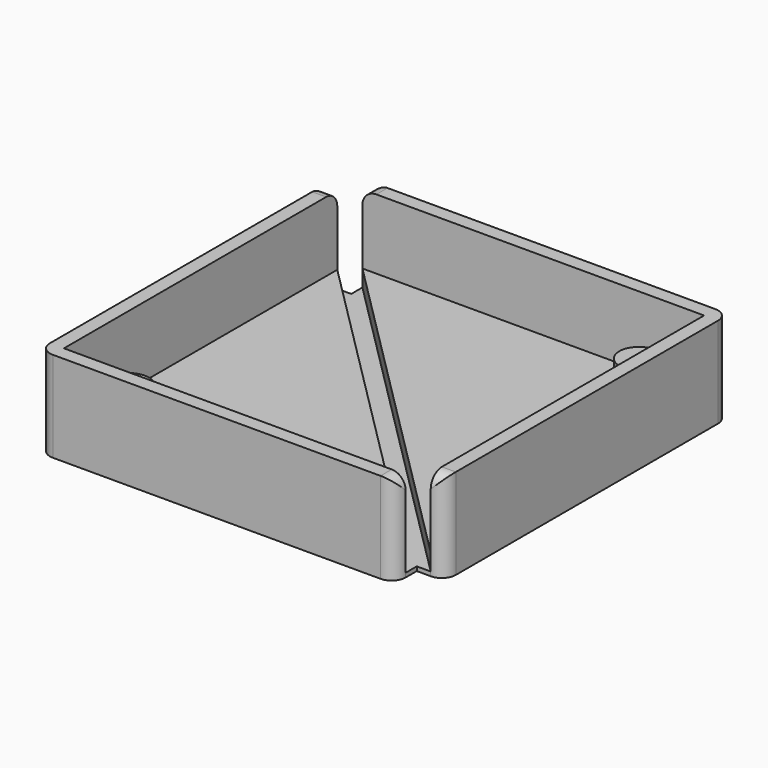
from build123d import *

# Parameters (mm, degrees)
F0_W     = 55
F0_H     = 55
F1_DEPTH = 3
F2_W     = 55
F2_H     = 55
F2_W_2   = 51
F2_H_2   = 51
F3_DEPTH = 10
F4_R     = 2.8
F5_DEPTH = 5
F6_W     = 4
F6_H     = 4
F7_DEPTH = 25
F9_DEPTH = 2.4
F10_R    = 1.99999


# Not quite as in the source:
# - a fillet or chamfer is up to 0.001 mm smaller than in the source, because OpenCascade refuses the exact size


with BuildPart() as f1:
    # F0 (on Top) → F1 (new body)
    with BuildSketch(Plane.XY):
        Rectangle(F0_W, F0_H)
    extrude(amount=F1_DEPTH)

    # F2 (on face) → F3 (join)
    with BuildSketch(Plane.XY.offset(3)):
        Rectangle(F2_W, F2_H)
        Rectangle(F2_W_2, F2_H_2, mode=Mode.SUBTRACT)
    extrude(amount=F3_DEPTH)

    # F4 (on face) → F5 (join)
    with BuildSketch(Plane.XY.offset(3)):
        with Locations((-20.3, -20.3)):
            Circle(F4_R)
        with Locations((20.3, 20.3)):
            Circle(F4_R)
    extrude(amount=F5_DEPTH)

    # F6 (on face) → F7 (cut)
    with BuildSketch(Plane.XY.offset(13)):
        with Locations((-25.5, 25.5)):
            Rectangle(F6_W, F6_H)
        with Locations((25.5, -25.5)):
            Rectangle(F6_W, F6_H)
    extrude(amount=-F7_DEPTH, mode=Mode.SUBTRACT)

    # F8 (on face) → F9 (cut)
    with BuildSketch(Plane.XY.offset(3)):
        Polygon((-23.5, 25.5), (-25.5, 23.5), (23.5, -25.5), (25.5, -23.5), align=None)
    extrude(amount=-F9_DEPTH, mode=Mode.SUBTRACT)

    # F10 (radius 2 in the source; OpenCascade refuses exactly that, so slightly less here)
    f10_edges = [f1.edges().sort_by_distance(p)[0] for p in [
        (-26.5, 23.5, 13),
        (23.5, -26.5, 13),
        (26.5, -23.5, 13),
        (-23.5, 26.5, 13),
        (-27.5, 23.5, 6.5),
        (-23.5, 27.5, 6.5),
        (23.5, -27.5, 6.5),
        (27.5, -23.5, 6.5),
        (-27.5, -27.5, 6.5),
        (27.5, 27.5, 6.5),
    ]]
    fillet(f10_edges, radius=F10_R)


solid = f1.part
